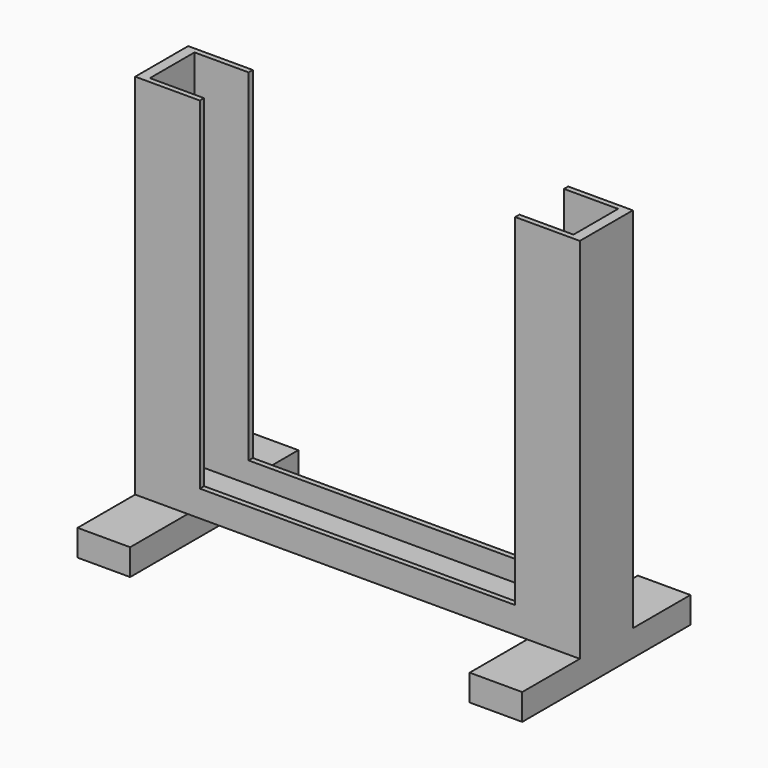
from build123d import *

# Parameters (mm, degrees)
F0_W     = 84.6
F0_H     = 70
F1_DEPTH = 6.3
F2_DEPTH = 6.3
F3_W     = 80.6
F3_H     = 10.6
F4_DEPTH = 69
F6_DEPTH = 25
F7_W     = 10
F7_H     = 40
F8_DEPTH = 5


# Not quite as in the source:
# - ends of sketch curves that miss each other by under 0.0002 mm in the source are joined


with BuildPart() as f1:
    # F0 (on Front) → F1 (new body)
    with BuildSketch(Plane.XZ):
        Rectangle(F0_W, F0_H)
    extrude(amount=F1_DEPTH)

    # F0 (on Front) → F2 (join)
    with BuildSketch(Plane.XZ):
        Rectangle(F0_W, F0_H)
    extrude(amount=-F2_DEPTH)

    # F3 (on face) → F4 (cut)
    with BuildSketch(Plane.XY.offset(35)):
        Rectangle(F3_W, F3_H)
    extrude(amount=-F4_DEPTH, mode=Mode.SUBTRACT)

    # F5 (on face) → F6 (cut)
    with BuildSketch(Plane.XZ.offset(6.3)):
        Polygon((-30, 30), (-30, -30), (30, -30), (30, 30), (30.0000030547, 35), (-30, 35), align=None)
    extrude(amount=-F6_DEPTH, mode=Mode.SUBTRACT)

    # F7 (on face) → F8 (join)
    with BuildSketch(Plane(origin=(0, 0, -35), x_dir=(1, 0, 0), z_dir=(0, 0, -1))):
        with Locations((-37.3, 0)):
            Rectangle(F7_W, F7_H)
        with Locations((37.3, 0)):
            Rectangle(F7_W, F7_H)
    extrude(amount=F8_DEPTH)


solid = f1.part
